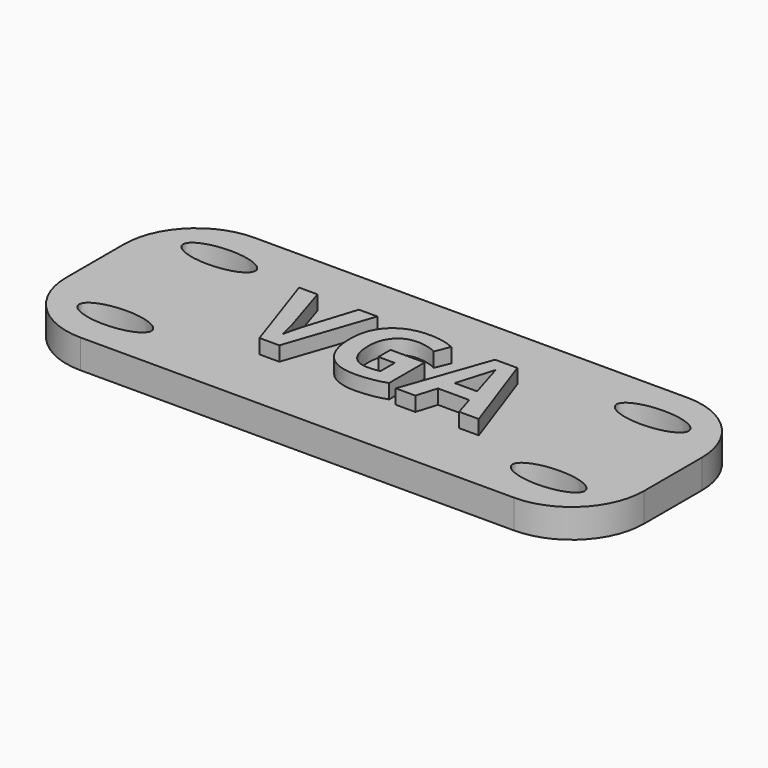
from build123d import *

# Parameters (mm, degrees)
F0_W         = 40
F0_H         = 15
F1_DEPTH     = 2
F2_TEXT_SIZE = 8.3333333333
F3_DEPTH     = 1
F4_R         = 5


# Not quite as in the source:
# - Text() gives the source's letters only with a copy of the font that has no kerning and outlines rounded to 1/6400 em; it was checked with that copy


with BuildPart() as f1:
    # F0 (on Top) → F1 (new body)
    with BuildSketch(Plane.XY):
        Rectangle(F0_W, F0_H)
        with BuildLine():
            add(Edge.make_bspline(
                [(-12.5, -4.5), (-12.5, -2.7679491924), (-16.25, -3.6339745962), (-20, -4.5), (-16.25, -5.3660254038), (-12.5, -6.2320508076), (-12.5, -4.5)],
                knots=[0, 0, 0, 2.0943951024, 2.0943951024, 4.1887902048, 4.1887902048, 6.2831853072, 6.2831853072, 6.2831853072], degree=2, weights=[1, 0.5, 1, 0.5, 1, 0.5, 1]))
        make_face(mode=Mode.SUBTRACT)
        with BuildLine():
            add(Edge.make_bspline(
                [(17.5, -4.5), (17.5, -2.7679491924), (13.75, -3.6339745962), (10, -4.5), (13.75, -5.3660254038), (17.5, -6.2320508076), (17.5, -4.5)],
                knots=[0, 0, 0, 2.0943951024, 2.0943951024, 4.1887902048, 4.1887902048, 6.2831853072, 6.2831853072, 6.2831853072], degree=2, weights=[1, 0.5, 1, 0.5, 1, 0.5, 1]))
        make_face(mode=Mode.SUBTRACT)
        with BuildLine():
            add(Edge.make_bspline(
                [(-12.5, 4.5), (-12.5, 6.2320508076), (-16.25, 5.3660254038), (-20, 4.5), (-16.25, 3.6339745962), (-12.5, 2.7679491924), (-12.5, 4.5)],
                knots=[0, 0, 0, 2.0943951024, 2.0943951024, 4.1887902048, 4.1887902048, 6.2831853072, 6.2831853072, 6.2831853072], degree=2, weights=[1, 0.5, 1, 0.5, 1, 0.5, 1]))
        make_face(mode=Mode.SUBTRACT)
        with BuildLine():
            add(Edge.make_bspline(
                [(17.5, 4.5), (17.5, 6.2320508076), (13.75, 5.3660254038), (10, 4.5), (13.75, 3.6339745962), (17.5, 2.7679491924), (17.5, 4.5)],
                knots=[0, 0, 0, 2.0943951024, 2.0943951024, 4.1887902048, 4.1887902048, 6.2831853072, 6.2831853072, 6.2831853072], degree=2, weights=[1, 0.5, 1, 0.5, 1, 0.5, 1]))
        make_face(mode=Mode.SUBTRACT)
    extrude(amount=F1_DEPTH)

    # F4
    f4_edges = [f1.edges().sort_by_distance(p)[0] for p in [
        (-20, -7.5, 1),
        (20, -7.5, 1),
        (20, 7.5, 1),
        (-20, 7.5, 1),
    ]]
    fillet(f4_edges, radius=F4_R)


with BuildPart() as f3:
    # F2 (on face) → F3 (new body)
    with BuildSketch(Plane.XY.offset(2)):
        with Locations((-8.2395833333, -3)):
            Text('VGA', F2_TEXT_SIZE, font='Open Sans', font_style=FontStyle.BOLD, text_align=(TextAlign.LEFT, TextAlign.BOTTOM))
    extrude(amount=F3_DEPTH)


solid = Compound([f1.part, f3.part])
